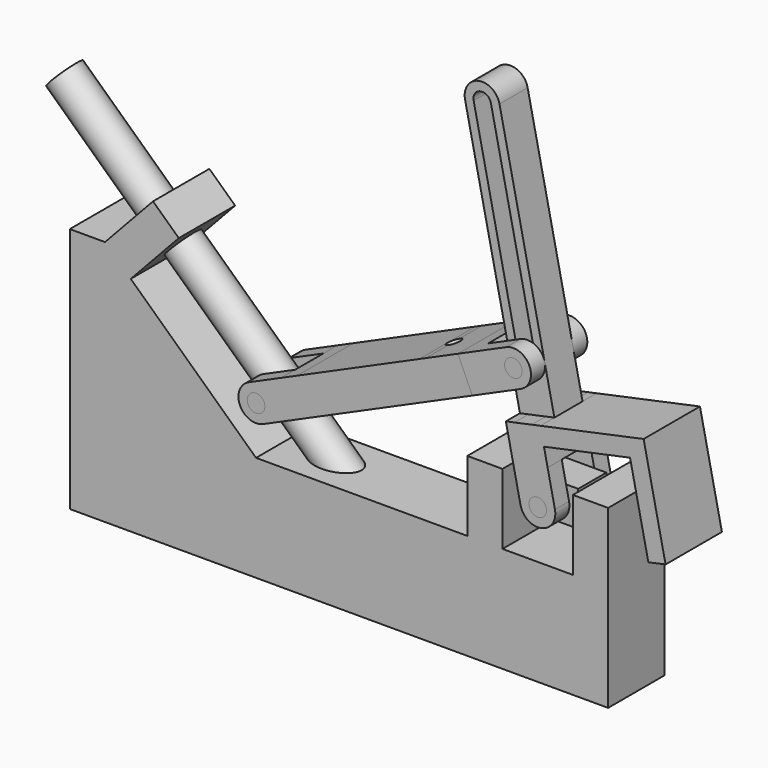
from build123d import *

# Parameters (mm, degrees)
F6_DEPTH  = 10
F8_DEPTH  = 12.5
F10_DEPTH = 10
F12_DEPTH = 10
F15_DEPTH = 5
F4_W      = 2.5
F4_H      = 2.5
F4_R      = 2.5
F17_DEPTH = 5
F19_DEPTH = 10
F20_DEPTH = 5
F21_DEPTH = 5
F22_DEPTH = 10


# Not quite as in the source:
# - a feature names something its author has since deleted; it is built from what else it names


with BuildPart() as f6:
    # F1 (on Front) → F6 (new body, symmetric)
    with BuildSketch(Plane.XZ):
        Polygon((60, -13.673274611), (0, -13.673274611), (-35.5812113848, 19.5067417884), (-21.9412441835, 34.1338158208), (-29.2547811997, 40.9537994214), (-42.894748401, 26.326725389), (-52.894748401, 26.326725389), (-52.894748401, -43.673274611), (70, -43.673274611), (100, -43.673274611), (100, -13.673274611), (100, 6.326725389), (90, 6.326725389), (90, -13.673274611), (70, -13.673274611), (70, 6.326725389), (60, 6.326725389), align=None)
    extrude(amount=F6_DEPTH, both=True)


with BuildPart() as f7:
    # F2 (on Front) → F7 (revolve)
    with BuildSketch(Plane.XZ):
        with BuildLine():
            Line((18.3197186482, -23.9200513188), (25.3864789566, -23.673274611))
            Line((25.3864789566, -23.673274611), (1.828384254, -1.7049959002))
            ThreePointArc((1.828384254, -1.7049959002), (-1.7049959002, -1.828384254), (-1.828384254, 1.7049959002))
            Line((-1.828384254, 1.7049959002), (-62.3759652377, 58.1665285965))
            Line((-62.3759652377, 58.1665285965), (-65.785957038, 54.5097600884))
            Line((-65.785957038, 54.5097600884), (18.3197186482, -23.9200513188))
        make_face()
        with BuildLine():
            ThreePointArc((-1.828384254, 1.7049959002), (-1.7049959002, -1.828384254), (1.828384254, -1.7049959002))
            Line((1.828384254, -1.7049959002), (-1.828384254, 1.7049959002))
        make_face()
    revolve(axis=Axis((-18.4947431405, 0, 17.2466269928), (-0.7313537016, 0, 0.6819983601)))

    # F2 (on Front) → F8 (cut, symmetric)
    with BuildSketch(Plane.XZ):
        with BuildLine():
            ThreePointArc((-1.828384254, 1.7049959002), (-1.7049959002, -1.828384254), (1.828384254, -1.7049959002))
            Line((1.828384254, -1.7049959002), (-1.828384254, 1.7049959002))
        make_face()
        with BuildLine():
            Line((-1.828384254, 1.7049959002), (1.828384254, -1.7049959002))
            ThreePointArc((1.828384254, -1.7049959002), (2.32604392, -0.9162530668), (2.5, 0))
            ThreePointArc((2.5, 0), (0.9162530668, 2.32604392), (-1.828384254, 1.7049959002))
        make_face()
    extrude(amount=F8_DEPTH, both=True, mode=Mode.SUBTRACT)


with BuildPart() as f6_1:
    add(f6.part)

    # F9: cut F7
    add(f7.part, mode=Mode.SUBTRACT)


with BuildPart() as f10:
    # F3 (on Front) → F10 (new body, symmetric)
    with BuildSketch(Plane.XZ):
        with BuildLine():
            Line((11.1691377918, -0.5003608575), (9.1354545764, 4.0673664308))
            Line((9.1354545764, 4.0673664308), (7.101771361, 8.635093719))
            Line((7.101771361, 8.635093719), (-2.0336832154, 4.5677272882))
            ThreePointArc((-2.0336832154, 4.5677272882), (-4.5677272882, -2.0336832154), (2.0336832154, -4.5677272882))
            Line((2.0336832154, -4.5677272882), (11.1691377918, -0.5003608575))
        make_face()
        with BuildLine():
            ThreePointArc((2.2838636441, 1.0168416077), (2.4453690018, 0.519779227), (2.5, 0))
            ThreePointArc((2.5, 0), (-2.4453690018, -0.519779227), (2.2838636441, 1.0168416077))
        make_face(mode=Mode.SUBTRACT)
        Polygon((7.101771361, 8.635093719), (9.1354545764, 4.0673664308), (13.7031818646, 6.1010496461), (11.6694986493, 10.6687769343), align=None)
        Polygon((13.7031818646, 6.1010496461), (9.1354545764, 4.0673664308), (11.1691377918, -0.5003608575), (15.73686508, 1.5333223579), align=None)
    extrude(amount=F10_DEPTH, both=True)

    # F3 (on Front) → F12 (join, symmetric)
    with BuildSketch(Plane.XZ):
        Polygon((11.6694986493, 10.6687769343), (13.7031818646, 6.1010496461), (45.6772728821, 20.3368321538), (45.0671679175, 21.7071503403), (44.6604312744, 22.6206957979), (47.4010676474, 23.8409057271), (46.3842260397, 26.1247693712), align=None)
        Polygon((45.6772728821, 20.3368321538), (13.7031818646, 6.1010496461), (15.73686508, 1.5333223579), (50.4515924704, 16.9893147948), (49.4347508627, 19.2731784389), (46.6941144898, 18.0529685097), (46.2873778467, 18.9665139673), align=None)
        Polygon((48.211316955, 26.9382426574), (46.3842260397, 26.1247693712), (47.4010676474, 23.8409057271), (49.2281585627, 24.6543790133), align=None)
        Polygon((47.4010676474, 23.8409057271), (47.8078042904, 22.9273602695), (49.6348952057, 23.7408335556), (49.2281585627, 24.6543790133), align=None)
        Polygon((49.6348952057, 23.7408335556), (58.7703497822, 27.8081999864), (58.3636131391, 28.721745444), (49.2281585627, 24.6543790133), align=None)
        Polygon((57.3467715314, 31.0056090881), (48.211316955, 26.9382426574), (49.2281585627, 24.6543790133), (58.3636131391, 28.721745444), align=None)
        Polygon((59.9905597114, 25.0675636135), (49.0280142197, 20.1867238966), (49.4347508627, 19.2731784389), (60.3972963545, 24.1540181558), align=None)
        Polygon((49.4347508627, 19.2731784389), (50.4515924704, 16.9893147948), (61.4141379621, 21.8701545117), (60.3972963545, 24.1540181558), align=None)
        Polygon((45.0671679175, 21.7071503403), (45.6772728821, 20.3368321538), (48.4179092551, 21.557042083), (47.8078042904, 22.9273602695), (47.4010676474, 23.8409057271), (44.6604312744, 22.6206957979), align=None)
        Polygon((48.4179092551, 21.557042083), (45.6772728821, 20.3368321538), (46.2873778467, 18.9665139673), (46.6941144898, 18.0529685097), (49.4347508627, 19.2731784389), (49.0280142197, 20.1867238966), align=None)
        Polygon((47.8078042904, 22.9273602695), (48.4179092551, 21.557042083), (59.3804547468, 26.4378817999), (58.7703497822, 27.8081999864), (49.6348952057, 23.7408335556), align=None)
        Polygon((59.3804547468, 26.4378817999), (48.4179092551, 21.557042083), (49.0280142197, 20.1867238966), (59.9905597114, 25.0675636135), align=None)
    extrude(amount=F12_DEPTH, both=True)

    # F3 (on Front) → F13 (revolve, cut)
    with BuildSketch(Plane.XZ):
        Polygon((45.0671679175, 21.7071503403), (45.6772728821, 20.3368321538), (48.4179092551, 21.557042083), (47.8078042904, 22.9273602695), (47.4010676474, 23.8409057271), (44.6604312744, 22.6206957979), align=None)
        Polygon((47.8078042904, 22.9273602695), (48.4179092551, 21.557042083), (59.3804547468, 26.4378817999), (58.7703497822, 27.8081999864), (49.6348952057, 23.7408335556), align=None)
        Polygon((47.4010676474, 23.8409057271), (47.8078042904, 22.9273602695), (49.6348952057, 23.7408335556), (49.2281585627, 24.6543790133), align=None)
        Polygon((49.6348952057, 23.7408335556), (58.7703497822, 27.8081999864), (58.3636131391, 28.721745444), (49.2281585627, 24.6543790133), align=None)
    revolve(axis=Axis((36.5418183057, 0, 16.269465723), (0.9135454576, 0, 0.4067366431)), mode=Mode.SUBTRACT)

    # F3 (on Front) → F14 (revolve, cut)
    with BuildSketch(Plane.XZ):
        Polygon((48.211316955, 26.9382426574), (46.3842260397, 26.1247693712), (47.4010676474, 23.8409057271), (49.2281585627, 24.6543790133), align=None)
        Polygon((47.4010676474, 23.8409057271), (47.8078042904, 22.9273602695), (49.6348952057, 23.7408335556), (49.2281585627, 24.6543790133), align=None)
    revolve(axis=Axis((48.9231060803, 0, 25.3395381065), (0.4067366431, 0, -0.9135454576)), mode=Mode.SUBTRACT)


with BuildPart() as f10b:
    # F3 (on Front) → F10, piece 2 (new body, symmetric)
    with BuildSketch(Plane.XZ):
        with BuildLine():
            Line((61.9144988196, 33.0392923035), (63.948182035, 28.4715650153))
            Line((63.948182035, 28.4715650153), (65.9818652504, 23.9038377271))
            Line((65.9818652504, 23.9038377271), (75.1173198268, 27.9712041579))
            ThreePointArc((75.1173198268, 27.9712041579), (77.6513638996, 34.5726146614), (71.049953396, 37.1066587343))
            Line((71.049953396, 37.1066587343), (61.9144988196, 33.0392923035))
        make_face()
        with BuildLine():
            ThreePointArc((75.5836366114, 32.5389314461), (73.6034158385, 30.0935624442), (70.7997729673, 31.5220898384))
            ThreePointArc((70.7997729673, 31.5220898384), (72.5638573844, 34.9843004479), (75.5836366114, 32.5389314461))
        make_face(mode=Mode.SUBTRACT)
        Polygon((58.7703497822, 27.8081999864), (59.3804547468, 26.4378817999), (63.948182035, 28.4715650153), (61.9144988196, 33.0392923035), (57.3467715314, 31.0056090881), (58.3636131391, 28.721745444), align=None)
        Polygon((63.948182035, 28.4715650153), (59.3804547468, 26.4378817999), (59.9905597114, 25.0675636135), (60.3972963545, 24.1540181558), (61.4141379621, 21.8701545117), (65.9818652504, 23.9038377271), align=None)
    extrude(amount=F10_DEPTH, both=True)

    # F3 (on Front) → F11 (revolve)
    with BuildSketch(Plane.XZ):
        Polygon((47.8078042904, 22.9273602695), (48.4179092551, 21.557042083), (59.3804547468, 26.4378817999), (58.7703497822, 27.8081999864), (49.6348952057, 23.7408335556), align=None)
        Polygon((45.0671679175, 21.7071503403), (45.6772728821, 20.3368321538), (48.4179092551, 21.557042083), (47.8078042904, 22.9273602695), (47.4010676474, 23.8409057271), (44.6604312744, 22.6206957979), align=None)
    revolve(axis=Axis((36.5418183057, 0, 16.269465723), (0.9135454576, 0, 0.4067366431)))


with BuildPart() as f15_tool:
    # F3 (on Front) → F15 (new body, symmetric)
    with BuildSketch(Plane.XZ):
        with BuildLine():
            Line((11.1691377918, -0.5003608575), (9.1354545764, 4.0673664308))
            Line((9.1354545764, 4.0673664308), (7.101771361, 8.635093719))
            Line((7.101771361, 8.635093719), (-2.0336832154, 4.5677272882))
            ThreePointArc((-2.0336832154, 4.5677272882), (-4.5677272882, -2.0336832154), (2.0336832154, -4.5677272882))
            Line((2.0336832154, -4.5677272882), (11.1691377918, -0.5003608575))
        make_face()
        with BuildLine():
            ThreePointArc((2.2838636441, 1.0168416077), (2.4453690018, 0.519779227), (2.5, 0))
            ThreePointArc((2.5, 0), (-2.4453690018, -0.519779227), (2.2838636441, 1.0168416077))
        make_face(mode=Mode.SUBTRACT)
        with BuildLine():
            Line((61.9144988196, 33.0392923035), (63.948182035, 28.4715650153))
            Line((63.948182035, 28.4715650153), (65.9818652504, 23.9038377271))
            Line((65.9818652504, 23.9038377271), (75.1173198268, 27.9712041579))
            ThreePointArc((75.1173198268, 27.9712041579), (77.6513638996, 34.5726146614), (71.049953396, 37.1066587343))
            Line((71.049953396, 37.1066587343), (61.9144988196, 33.0392923035))
        make_face()
        with BuildLine():
            ThreePointArc((75.5836366114, 32.5389314461), (73.6034158385, 30.0935624442), (70.7997729673, 31.5220898384))
            ThreePointArc((70.7997729673, 31.5220898384), (72.5638573844, 34.9843004479), (75.5836366114, 32.5389314461))
        make_face(mode=Mode.SUBTRACT)
    extrude(amount=F15_DEPTH, both=True)


with BuildPart() as f10_1:
    add(f10.part)

    # F15: cut by f15_tool
    add(f15_tool.part, mode=Mode.SUBTRACT)


with BuildPart() as f10b_1:
    add(f10b.part)

    # F15: cut by f15_tool
    add(f15_tool.part, mode=Mode.SUBTRACT)


with BuildPart() as f16:
    # F4 (on Front) → F16 (revolve)
    with BuildSketch(Plane.XZ):
        with Locations((71.25, 1.25)):
            Rectangle(F4_W, F4_H)
        with Locations((68.75, 1.25)):
            Rectangle(F4_W, F4_H)
    revolve(axis=Axis((70, 0, 0), (-1, 0, 0)))



with BuildPart() as f16b:
    # F4 (on Front) → F16, piece 2 (revolve)
    with BuildSketch(Plane.XZ):
        with Locations((88.75, 1.25)):
            Rectangle(F4_W, F4_H)
        with Locations((91.25, 1.25)):
            Rectangle(F4_W, F4_H)
    revolve(axis=Axis((70, 0, 0), (-1, 0, 0)))


with BuildPart() as f16_1:
    add(f16.part)

    add(f16b.part)  # F17 merges F16b
    # F4 (on Front) → F17 (join, symmetric)
    with BuildSketch(Plane.XZ):
        Polygon((72.5, 0), (72.5, -2.5), (72.5, -5), (87.5, -5), (87.5, -2.5), (87.5, 0), (87.5, 2.5), (87.5, 5), (72.5, 5), (72.5, 2.5), align=None)
        with Locations((80, 0)):
            Circle(F4_R, mode=Mode.SUBTRACT)
    extrude(amount=F17_DEPTH, both=True)


with BuildPart() as f6_2:
    add(f6_1.part)

    # F18: cut F16
    add(f16_1.part, mode=Mode.SUBTRACT)


with BuildPart() as f19:
    # F5 (on Front) → F19 (new body, symmetric)
    with BuildSketch(Plane.XZ):
        with BuildLine():
            Line((80.3662520937, 10.3012552344), (81.5450849719, 4.7552825815))
            ThreePointArc((81.5450849719, 4.7552825815), (83.7157241274, 3.3456530318), (84.8907380037, 1.0395584541))
            Line((84.8907380037, 1.0395584541), (82.8116210955, 10.8210344614))
            Line((82.8116210955, 10.8210344614), (80.3662520937, 10.3012552344))
        make_face()
        with BuildLine():
            ThreePointArc((76.6543469682, 3.7157241274), (78.9604415459, 4.8907380037), (81.5450849719, 4.7552825815))
            Line((81.5450849719, 4.7552825815), (80.3662520937, 10.3012552344))
            Line((80.3662520937, 10.3012552344), (75.47551409, 9.2616967803))
            Line((75.47551409, 9.2616967803), (76.6543469682, 3.7157241274))
        make_face()
        with BuildLine():
            ThreePointArc((75.1092619963, -1.0395584541), (75.2447174185, 1.5450849719), (76.6543469682, 3.7157241274))
            Line((76.6543469682, 3.7157241274), (75.47551409, 9.2616967803))
            Line((75.47551409, 9.2616967803), (73.0301450882, 8.7419175532))
            Line((73.0301450882, 8.7419175532), (75.1092619963, -1.0395584541))
        make_face()
        with BuildLine():
            ThreePointArc((82.4453690018, 0.519779227), (82.4863047384, 0.2613211582), (82.5, 0))
            ThreePointArc((82.5, 0), (80.2613211582, -2.4863047384), (77.5546309982, -0.519779227))
            Line((77.5546309982, -0.519779227), (76.6543469682, 3.7157241274))
            ThreePointArc((76.6543469682, 3.7157241274), (75.2447174185, 1.5450849719), (75.1092619963, -1.0395584541))
            ThreePointArc((75.1092619963, -1.0395584541), (80.5226423163, -4.9726094768), (85, 0))
            ThreePointArc((85, 0), (84.9726094768, 0.5226423163), (84.8907380037, 1.0395584541))
            ThreePointArc((84.8907380037, 1.0395584541), (83.7157241274, 3.3456530318), (81.5450849719, 4.7552825815))
            Line((81.5450849719, 4.7552825815), (82.4453690018, 0.519779227))
        make_face()
        with BuildLine():
            ThreePointArc((77.5546309982, -0.519779227), (79.480220773, 2.4453690018), (82.4453690018, 0.519779227))
            Line((82.4453690018, 0.519779227), (81.5450849719, 4.7552825815))
            ThreePointArc((81.5450849719, 4.7552825815), (78.9604415459, 4.8907380037), (76.6543469682, 3.7157241274))
            Line((76.6543469682, 3.7157241274), (77.5546309982, -0.519779227))
        make_face()
        Polygon((75.47551409, 9.2616967803), (80.3662520937, 10.3012552344), (78.2871351855, 20.0827312417), (73.3963971818, 19.0431727876), align=None)
        Polygon((73.0301450882, 8.7419175532), (75.47551409, 9.2616967803), (73.3963971818, 19.0431727876), (70.95102818, 18.5233935606), align=None)
        Polygon((78.2871351855, 20.0827312417), (80.3662520937, 10.3012552344), (82.8116210955, 10.8210344614), (81.7720630055, 15.711770752), (106.2257513108, 20.9095626583), (111.4235432171, -3.5441256469), (116.3142829339, -2.5045668287), (110.0769322093, 26.8398611933), (80.7325041873, 20.6025104688), align=None)
    extrude(amount=F19_DEPTH, both=True)

    # F5 (on Front) → F20 (join, symmetric)
    with BuildSketch(Plane.XZ):
        with BuildLine():
            Line((75.5290056132, 33.0587106731), (78.2871351855, 20.0827312417))
            Line((78.2871351855, 20.0827312417), (80.7325041873, 20.6025104688))
            Line((80.7325041873, 20.6025104688), (65.139127376, 93.9635805238))
            ThreePointArc((65.139127376, 93.9635805238), (59.2088309182, 97.8147600734), (55.3576513686, 91.8844636156))
            Line((55.3576513686, 91.8844636156), (70.95102818, 18.5233935606))
            Line((70.95102818, 18.5233935606), (73.3963971818, 19.0431727876))
            Line((73.3963971818, 19.0431727876), (70.6382676096, 32.019152219))
            Line((70.6382676096, 32.019152219), (57.8030203705, 92.4042428427))
            ThreePointArc((57.8030203705, 92.4042428427), (59.7286101453, 95.3693910715), (62.6937583741, 93.4438012968))
            Line((62.6937583741, 93.4438012968), (75.5290056132, 33.0587106731))
        make_face()
        with BuildLine():
            Line((73.3963971818, 19.0431727876), (78.2871351855, 20.0827312417))
            Line((78.2871351855, 20.0827312417), (75.5290056132, 33.0587106731))
            ThreePointArc((75.5290056132, 33.0587106731), (73.6034158385, 30.0935624442), (70.6382676096, 32.019152219))
            Line((70.6382676096, 32.019152219), (73.3963971818, 19.0431727876))
        make_face()
    extrude(amount=F20_DEPTH, both=True)

    # F5 (on Front) → F21 (cut, symmetric)
    with BuildSketch(Plane.XZ):
        with BuildLine():
            ThreePointArc((76.6543469682, 3.7157241274), (78.9604415459, 4.8907380037), (81.5450849719, 4.7552825815))
            Line((81.5450849719, 4.7552825815), (80.3662520937, 10.3012552344))
            Line((80.3662520937, 10.3012552344), (75.47551409, 9.2616967803))
            Line((75.47551409, 9.2616967803), (76.6543469682, 3.7157241274))
        make_face()
        with BuildLine():
            Line((80.3662520937, 10.3012552344), (81.5450849719, 4.7552825815))
            ThreePointArc((81.5450849719, 4.7552825815), (83.7157241274, 3.3456530318), (84.8907380037, 1.0395584541))
            Line((84.8907380037, 1.0395584541), (82.8116210955, 10.8210344614))
            Line((82.8116210955, 10.8210344614), (80.3662520937, 10.3012552344))
        make_face()
        with BuildLine():
            ThreePointArc((75.1092619963, -1.0395584541), (75.2447174185, 1.5450849719), (76.6543469682, 3.7157241274))
            Line((76.6543469682, 3.7157241274), (75.47551409, 9.2616967803))
            Line((75.47551409, 9.2616967803), (73.0301450882, 8.7419175532))
            Line((73.0301450882, 8.7419175532), (75.1092619963, -1.0395584541))
        make_face()
        with BuildLine():
            ThreePointArc((82.4453690018, 0.519779227), (82.4863047384, 0.2613211582), (82.5, 0))
            ThreePointArc((82.5, 0), (80.2613211582, -2.4863047384), (77.5546309982, -0.519779227))
            Line((77.5546309982, -0.519779227), (76.6543469682, 3.7157241274))
            ThreePointArc((76.6543469682, 3.7157241274), (75.2447174185, 1.5450849719), (75.1092619963, -1.0395584541))
            ThreePointArc((75.1092619963, -1.0395584541), (80.5226423163, -4.9726094768), (85, 0))
            ThreePointArc((85, 0), (84.9726094768, 0.5226423163), (84.8907380037, 1.0395584541))
            ThreePointArc((84.8907380037, 1.0395584541), (83.7157241274, 3.3456530318), (81.5450849719, 4.7552825815))
            Line((81.5450849719, 4.7552825815), (82.4453690018, 0.519779227))
        make_face()
        with BuildLine():
            ThreePointArc((77.5546309982, -0.519779227), (79.480220773, 2.4453690018), (82.4453690018, 0.519779227))
            Line((82.4453690018, 0.519779227), (81.5450849719, 4.7552825815))
            ThreePointArc((81.5450849719, 4.7552825815), (78.9604415459, 4.8907380037), (76.6543469682, 3.7157241274))
            Line((76.6543469682, 3.7157241274), (77.5546309982, -0.519779227))
        make_face()
    extrude(amount=F21_DEPTH, both=True, mode=Mode.SUBTRACT)


with BuildPart() as f22:
    # F2 (on Front) → F22 (new body, symmetric)
    with BuildSketch(Plane.XZ):
        with BuildLine():
            ThreePointArc((-1.828384254, 1.7049959002), (-1.7049959002, -1.828384254), (1.828384254, -1.7049959002))
            Line((1.828384254, -1.7049959002), (-1.828384254, 1.7049959002))
        make_face()
        with BuildLine():
            Line((-1.828384254, 1.7049959002), (1.828384254, -1.7049959002))
            ThreePointArc((1.828384254, -1.7049959002), (2.32604392, -0.9162530668), (2.5, 0))
            ThreePointArc((2.5, 0), (0.9162530668, 2.32604392), (-1.828384254, 1.7049959002))
        make_face()
    extrude(amount=F22_DEPTH, both=True)


with BuildPart() as f22b:
    # F5 (on Front) → F22, piece 2 (new body, symmetric)
    with BuildSketch(Plane.XZ):
        with BuildLine():
            ThreePointArc((77.5546309982, -0.519779227), (80.2613211582, -2.4863047384), (82.5, 0))
            ThreePointArc((82.5, 0), (82.4863047384, 0.2613211582), (82.4453690018, 0.519779227))
            ThreePointArc((82.4453690018, 0.519779227), (79.480220773, 2.4453690018), (77.5546309982, -0.519779227))
        make_face()
    extrude(amount=F22_DEPTH, both=True)


with BuildPart() as f22c:
    # F3 (on Front) → F22, piece 3 (new body, symmetric)
    with BuildSketch(Plane.XZ):
        with BuildLine():
            ThreePointArc((75.5836366114, 32.5389314461), (72.5638573844, 34.9843004479), (70.7997729673, 31.5220898384))
            ThreePointArc((70.7997729673, 31.5220898384), (73.6034158385, 30.0935624442), (75.5836366114, 32.5389314461))
        make_face()
    extrude(amount=F22_DEPTH, both=True)


solid = Compound([f7.part, f10_1.part, f10b_1.part, f16_1.part, f6_2.part, f19.part, f22.part, f22b.part, f22c.part])
